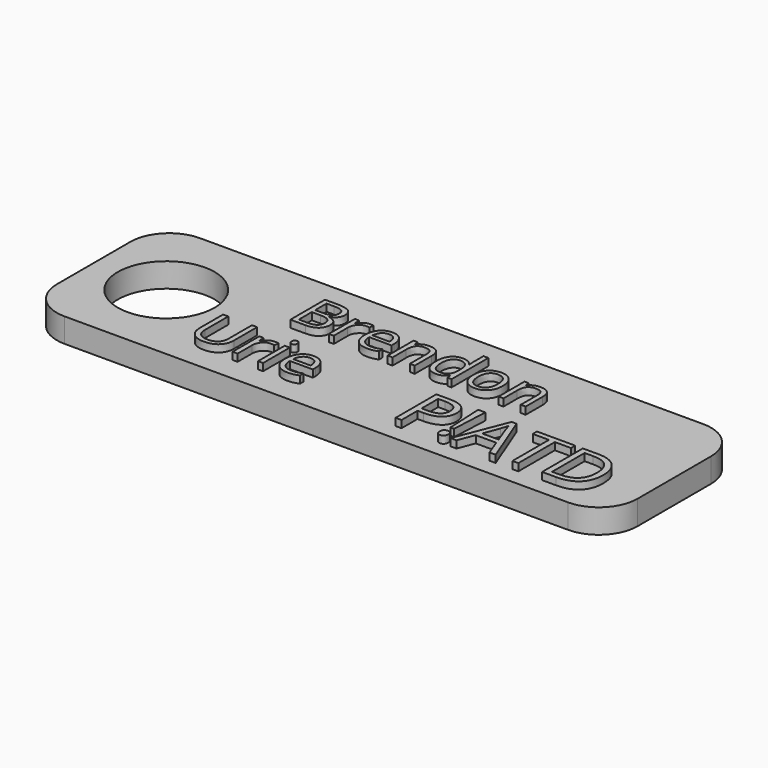
from build123d import *

# Parameters (mm, degrees)
F0_W           = 120
F0_H           = 35
F0_R           = 10
F1_DEPTH       = 5
F2_R           = 8
F4_TEXT_SIZE   = 12.5210431482
F4_TEXT_SIZE_2 = 12.8893097604
F4_TEXT_SIZE_3 = 14.7306402343
F5_DEPTH       = 1.5


# Not quite as in the source:
# - Text() gives the source's letters only with a copy of the font that has no kerning and outlines rounded to 1/6400 em; it was checked with that copy


with BuildPart() as f1:
    # F0 (on Top) → F1 (new body)
    with BuildSketch(Plane.XY):
        Rectangle(F0_W, F0_H)
        with Locations((-45, 0)):
            Circle(F0_R, mode=Mode.SUBTRACT)
    extrude(amount=F1_DEPTH)

    # F2
    f2_edges = [f1.edges().sort_by_distance(p)[0] for p in [
        (-60, 17.5, 2.5),
        (60, 17.5, 2.5),
        (60, -17.5, 2.5),
        (-60, -17.5, 2.5),
    ]]
    fillet(f2_edges, radius=F2_R)

    # F4 (on face) → F5 (join)
    with BuildSketch(Plane.XY.offset(5)):
        with Locations((-22.2727283835, 2.1212121937)):
            Text('Brendon', F4_TEXT_SIZE, font='Open Sans', text_align=(TextAlign.LEFT, TextAlign.BOTTOM))
        with Locations((-31.8181850016, -12.4621214345)):
            Text('Urie', F4_TEXT_SIZE_2, font='Open Sans', text_align=(TextAlign.LEFT, TextAlign.BOTTOM))
        with Locations((12.1969701722, -14.0530308709)):
            Text('P!ATD', F4_TEXT_SIZE_3, font='Open Sans', text_align=(TextAlign.LEFT, TextAlign.BOTTOM))
    extrude(amount=F5_DEPTH)


solid = f1.part
